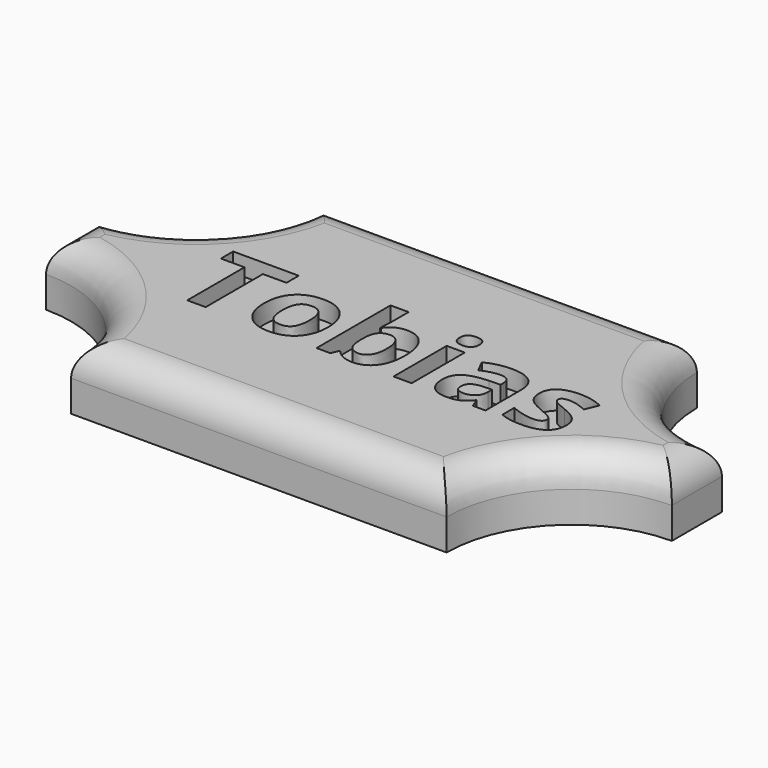
from build123d import *

# Parameters (mm, degrees)
F1_DEPTH     = 10
F2_R         = 5
F3_TEXT_SIZE = 19.4444444444
F4_DEPTH     = 3


# Not quite as in the source:
# - Text() gives the source's letters only with a copy of the font that has no kerning and outlines rounded to 1/6400 em; it was checked with that copy


with BuildPart() as f1:
    # F0 (on Top) → F1 (new body)
    with BuildSketch(Plane.XY):
        with BuildLine():
            ThreePointArc((0, 20), (14.1421356237, 14.1421356237), (20, 0))
            Line((20, 0), (80, 0))
            ThreePointArc((80, 0), (85.8578643763, 14.1421356237), (100, 20))
            Line((100, 20), (100, 30))
            ThreePointArc((100, 30), (85.8578643763, 35.8578643763), (80, 50))
            Line((80, 50), (20, 50))
            ThreePointArc((20, 50), (14.1421356237, 35.8578643763), (0, 30))
            Line((0, 30), (0, 20))
        make_face()
    extrude(amount=F1_DEPTH)

    # F2
    f2_edges = [f1.edges().sort_by_distance(p)[0] for p in [
        (50, 0, 10),
        (14.142136, 14.142136, 10),
        (0, 25, 10),
        (14.142136, 35.857864, 10),
        (50, 50, 10),
        (85.857864, 35.857864, 10),
        (85.857864, 14.142136, 10),
        (100, 25, 10),
    ]]
    fillet(f2_edges, radius=F2_R)

    # F3 (on face) → F4 (cut)
    with BuildSketch(Plane.XY.offset(10)):
        with Locations((20, 18)):
            Text('Tobias', F3_TEXT_SIZE, font='Open Sans', font_style=FontStyle.BOLD, text_align=(TextAlign.LEFT, TextAlign.BOTTOM))
    extrude(amount=-F4_DEPTH, mode=Mode.SUBTRACT)


solid = f1.part
